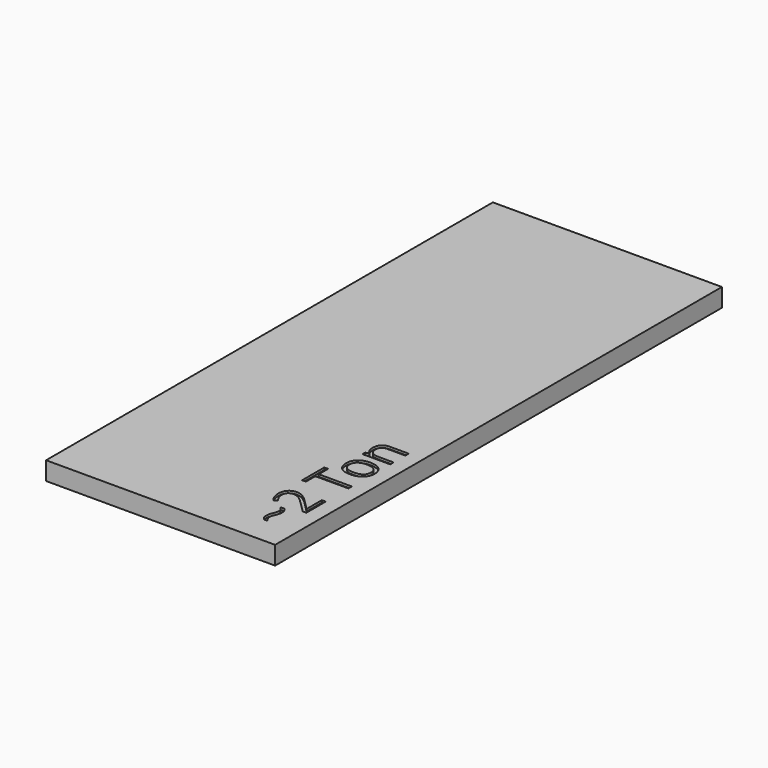
from build123d import *

# Parameters (mm, degrees)
F0_W         = 2500
F0_H         = 6096
F0_TEXT_SIZE = 565.0795168347
F1_DEPTH     = 200
F2_DEPTH     = 25


# Not quite as in the source:
# - Text() gives the source's letters only with a copy of the font that has no kerning and outlines rounded to 1/6400 em; it was checked with that copy


with BuildPart() as f1:
    # F0 (on Top) → F1 (new body)
    with BuildSketch(Plane.XY):
        Rectangle(F0_W, F0_H)
        with BuildLine():
            add(Edge.make_bspline(
                [(894.5491941284, -2651.680302651), (891.2381813344, -2664.1297107562), (891.2381813344, -2677.3737619321)],
                knots=[0, 0, 0, 1, 1, 1], degree=2))
            add(Edge.make_bspline(
                [(891.2381813344, -2677.3737619321), (891.2381813344, -2691.9422182254), (900.4648703202, -2709.4685126148)],
                knots=[0, 0, 0, 1, 1, 1], degree=2))
            add(Edge.make_bspline(
                [(900.4648703202, -2709.4685126148), (909.691559306, -2726.9948070041), (924.6131902975, -2741.9164379955)],
                knots=[0, 0, 0, 1, 1, 1], degree=2))
            Line((924.6131902975, -2741.9164379955), (882.9385759309, -2741.9164379955))
            add(Edge.make_bspline(
                [(882.9385759309, -2741.9164379955), (852.8304329245, -2714.2805178753), (852.8304329245, -2674.5483643479)],
                knots=[0, 0, 0, 1, 1, 1], degree=2))
            add(Edge.make_bspline(
                [(852.8304329245, -2674.5483643479), (852.8304329245, -2655.8301053527), (856.7153546028, -2640.2462718025)],
                knots=[0, 0, 0, 1, 1, 1], degree=2))
            add(Edge.make_bspline(
                [(856.7153546028, -2640.2462718025), (860.600276281, -2624.6624382523), (871.1072235472, -2600.1167967398)],
                knots=[0, 0, 0, 1, 1, 1], degree=2))
            add(Edge.make_bspline(
                [(871.1072235472, -2600.1167967398), (878.7887732291, -2581.8400061172), (882.5412543956, -2568.3310739179)],
                knots=[0, 0, 0, 1, 1, 1], degree=2))
            add(Edge.make_bspline(
                [(882.5412543956, -2568.3310739179), (886.2937355621, -2554.8221417185), (886.2937355621, -2541.8429715662)],
                knots=[0, 0, 0, 1, 1, 1], degree=2))
            add(Edge.make_bspline(
                [(886.2937355621, -2541.8429715662), (886.2937355621, -2527.0096342493), (877.4643681116, -2509.3508993482)],
                knots=[0, 0, 0, 1, 1, 1], degree=2))
            add(Edge.make_bspline(
                [(877.4643681116, -2509.3508993482), (868.635000661, -2491.6921644472), (852.8304329245, -2476.7705334557)],
                knots=[0, 0, 0, 1, 1, 1], degree=2))
            Line((852.8304329245, -2476.7705334557), (894.2401662676, -2476.7705334557))
            add(Edge.make_bspline(
                [(894.2401662676, -2476.7705334557), (924.6131902975, -2504.936215623), (924.6131902975, -2544.0503134289)],
                knots=[0, 0, 0, 1, 1, 1], degree=2))
            add(Edge.make_bspline(
                [(924.6131902975, -2544.0503134289), (924.6131902975, -2563.9163901926), (920.0660660604, -2581.3102440702)],
                knots=[0, 0, 0, 1, 1, 1], degree=2))
            add(Edge.make_bspline(
                [(920.0660660604, -2581.3102440702), (915.5189418234, -2598.7040979477), (906.6895743729, -2618.5701747114)],
                knots=[0, 0, 0, 1, 1, 1], degree=2))
            add(Edge.make_bspline(
                [(906.6895743729, -2618.5701747114), (897.8602069223, -2639.2308945457), (894.5491941284, -2651.680302651)],
                knots=[0, 0, 0, 1, 1, 1], degree=2))
        make_face(mode=Mode.SUBTRACT)
        with BuildLine():
            Line((1045.4872306954, -2154.7635025345), (1087.9564881325, -2154.7635025345))
            Line((1087.9564881325, -2154.7635025345), (1087.9564881325, -2419.9094070743))
            Line((1087.9564881325, -2419.9094070743), (1048.4892156286, -2419.9094070743))
            Line((1048.4892156286, -2419.9094070743), (941.7421631515, -2313.6921166442))
            add(Edge.make_bspline(
                [(941.7421631515, -2313.6921166442), (892.562586452, -2265.1305956663), (871.5928387569, -2249.6792026278)],
                knots=[0, 0, 0, 1, 1, 1], degree=2))
            add(Edge.make_bspline(
                [(871.5928387569, -2249.6792026278), (850.6230910619, -2234.2278095894), (830.7570142982, -2226.5021130701)],
                knots=[0, 0, 0, 1, 1, 1], degree=2))
            add(Edge.make_bspline(
                [(830.7570142982, -2226.5021130701), (810.8909375345, -2218.7764165509), (788.0228758376, -2218.7764165509)],
                knots=[0, 0, 0, 1, 1, 1], degree=2))
            add(Edge.make_bspline(
                [(788.0228758376, -2218.7764165509), (755.7073909686, -2218.7764165509), (736.8125446244, -2238.3776122911)],
                knots=[0, 0, 0, 1, 1, 1], degree=2))
            add(Edge.make_bspline(
                [(736.8125446244, -2238.3776122911), (717.9176982803, -2257.9788080313), (717.9176982803, -2292.7665157864)],
                knots=[0, 0, 0, 1, 1, 1], degree=2))
            add(Edge.make_bspline(
                [(717.9176982803, -2292.7665157864), (717.9176982803, -2317.841919346), (726.2173036838, -2340.3568063449)],
                knots=[0, 0, 0, 1, 1, 1], degree=2))
            add(Edge.make_bspline(
                [(726.2173036838, -2340.3568063449), (734.5169090873, -2362.8716933438), (756.3254466901, -2390.4193197894)],
                knots=[0, 0, 0, 1, 1, 1], degree=2))
            Line((756.3254466901, -2390.4193197894), (725.1577795897, -2414.7000802784))
            add(Edge.make_bspline(
                [(725.1577795897, -2414.7000802784), (678.8036004744, -2358.9867716655), (678.8036004744, -2293.2962778335)],
                knots=[0, 0, 0, 1, 1, 1], degree=2))
            add(Edge.make_bspline(
                [(678.8036004744, -2293.2962778335), (678.8036004744, -2236.435151452), (707.8963662239, -2204.1638134203)],
                knots=[0, 0, 0, 1, 1, 1], degree=2))
            add(Edge.make_bspline(
                [(707.8963662239, -2204.1638134203), (736.9891319734, -2171.8924753885), (786.0804149984, -2171.8924753885)],
                knots=[0, 0, 0, 1, 1, 1], degree=2))
            add(Edge.make_bspline(
                [(786.0804149984, -2171.8924753885), (824.4881634083, -2171.8924753885), (862.0129750731, -2193.4361319679)],
                knots=[0, 0, 0, 1, 1, 1], degree=2))
            add(Edge.make_bspline(
                [(862.0129750731, -2193.4361319679), (899.5377867379, -2214.9797885472), (956.9286751664, -2273.9599631168)],
                knots=[0, 0, 0, 1, 1, 1], degree=2))
            Line((956.9286751664, -2273.9599631168), (1043.2798888327, -2362.2536376222))
            Line((1043.2798888327, -2362.2536376222), (1045.4872306954, -2362.2536376222))
            Line((1045.4872306954, -2362.2536376222), (1045.4872306954, -2154.7635025345))
        make_face(mode=Mode.SUBTRACT)
        Polygon((726.2173036838, -1798.0570575326), (1087.9564881325, -1798.0570575326), (1087.9564881325, -1844.940998695), (726.2173036838, -1844.940998695), (726.2173036838, -1972.7019457043), (684.5426893172, -1972.7019457043), (684.5426893172, -1670.2961105232), (726.2173036838, -1670.2961105232), align=None, mode=Mode.SUBTRACT)
        with BuildLine():
            add(Edge.make_bspline(
                [(822.2366747084, -1392.83323839), (864.4851979593, -1355.4408672369), (936.4445426812, -1355.4408672369)],
                knots=[0, 0, 0, 1, 1, 1], degree=2))
            add(Edge.make_bspline(
                [(936.4445426812, -1355.4408672369), (1010.4346419167, -1355.4408672369), (1051.9768157715, -1392.656651041)],
                knots=[0, 0, 0, 1, 1, 1], degree=2))
            add(Edge.make_bspline(
                [(1051.9768157715, -1392.656651041), (1093.5189896263, -1429.872434845), (1093.5189896263, -1495.562928677)],
                knots=[0, 0, 0, 1, 1, 1], degree=2))
            add(Edge.make_bspline(
                [(1093.5189896263, -1495.562928677), (1093.5189896263, -1536.1780189495), (1074.4475559331, -1567.6105670734)],
                knots=[0, 0, 0, 1, 1, 1], degree=2))
            add(Edge.make_bspline(
                [(1074.4475559331, -1567.6105670734), (1055.37612224, -1599.0431151974), (1019.7937714143, -1616.1720880514)],
                knots=[0, 0, 0, 1, 1, 1], degree=2))
            add(Edge.make_bspline(
                [(1019.7937714143, -1616.1720880514), (984.2114205886, -1633.3010609055), (936.4445426812, -1633.3010609055)],
                knots=[0, 0, 0, 1, 1, 1], degree=2))
            add(Edge.make_bspline(
                [(936.4445426812, -1633.3010609055), (862.5427371201, -1633.3010609055), (821.2654442889, -1596.3060112877)],
                knots=[0, 0, 0, 1, 1, 1], degree=2))
            add(Edge.make_bspline(
                [(821.2654442889, -1596.3060112877), (779.9881514576, -1559.3109616699), (779.9881514576, -1493.6204678379)],
                knots=[0, 0, 0, 1, 1, 1], degree=2))
            add(Edge.make_bspline(
                [(779.9881514576, -1493.6204678379), (779.9881514576, -1430.225609543), (822.2366747084, -1392.83323839)],
                knots=[0, 0, 0, 1, 1, 1], degree=2))
        make_face(mode=Mode.SUBTRACT)
        with BuildLine():
            Line((1087.9564881325, -1022.308833328), (1087.9564881325, -1068.1332503963))
            Line((1087.9564881325, -1068.1332503963), (892.2977054285, -1068.1332503963))
            add(Edge.make_bspline(
                [(892.2977054285, -1068.1332503963), (855.3909494852, -1068.1332503963), (837.1583056998, -1084.9531953896)],
                knots=[0, 0, 0, 1, 1, 1], degree=2))
            add(Edge.make_bspline(
                [(837.1583056998, -1084.9531953896), (818.9256619145, -1101.7731403828), (818.9256619145, -1137.7086659066)],
                knots=[0, 0, 0, 1, 1, 1], degree=2))
            add(Edge.make_bspline(
                [(818.9256619145, -1137.7086659066), (818.9256619145, -1185.122369116), (844.5749743583, -1207.1957877423)],
                knots=[0, 0, 0, 1, 1, 1], degree=2))
            add(Edge.make_bspline(
                [(844.5749743583, -1207.1957877423), (870.2242868021, -1229.2692063687), (929.2927550462, -1229.2692063687)],
                knots=[0, 0, 0, 1, 1, 1], degree=2))
            Line((929.2927550462, -1229.2692063687), (1087.9564881325, -1229.2692063687))
            Line((1087.9564881325, -1229.2692063687), (1087.9564881325, -1275.093623437))
            Line((1087.9564881325, -1275.093623437), (785.5506529514, -1275.093623437))
            Line((785.5506529514, -1275.093623437), (785.5506529514, -1237.8336927957))
            Line((785.5506529514, -1237.8336927957), (826.9603862945, -1230.4170241372))
            Line((826.9603862945, -1230.4170241372), (826.9603862945, -1228.2096822746))
            add(Edge.make_bspline(
                [(826.9603862945, -1228.2096822746), (804.6220866446, -1214.0826943537), (792.3051190511, -1188.6982629334)],
                knots=[0, 0, 0, 1, 1, 1], degree=2))
            add(Edge.make_bspline(
                [(792.3051190511, -1188.6982629334), (779.9881514576, -1163.3138315131), (779.9881514576, -1132.1461644127)],
                knots=[0, 0, 0, 1, 1, 1], degree=2))
            add(Edge.make_bspline(
                [(779.9881514576, -1132.1461644127), (779.9881514576, -1077.4923798939), (806.3438132974, -1049.9006066109)],
                knots=[0, 0, 0, 1, 1, 1], degree=2))
            add(Edge.make_bspline(
                [(806.3438132974, -1049.9006066109), (832.6994751373, -1022.308833328), (890.7084192874, -1022.308833328)],
                knots=[0, 0, 0, 1, 1, 1], degree=2))
            Line((890.7084192874, -1022.308833328), (1087.9564881325, -1022.308833328))
        make_face(mode=Mode.SUBTRACT)
        with BuildLine():
            add(Edge.make_bspline(
                [(848.4598960365, -1562.8868554874), (877.9941301586, -1585.7990640216), (936.4445426812, -1585.7990640216)],
                knots=[0, 0, 0, 1, 1, 1], degree=2))
            add(Edge.make_bspline(
                [(936.4445426812, -1585.7990640216), (994.4534868312, -1585.7990640216), (1024.7823640238, -1562.6219744639)],
                knots=[0, 0, 0, 1, 1, 1], degree=2))
            add(Edge.make_bspline(
                [(1024.7823640238, -1562.6219744639), (1055.1112412165, -1539.4448849062), (1055.1112412165, -1494.503404583)],
                knots=[0, 0, 0, 1, 1, 1], degree=2))
            add(Edge.make_bspline(
                [(1055.1112412165, -1494.503404583), (1055.1112412165, -1449.4736305852), (1024.9148045356, -1426.1641005158)],
                knots=[0, 0, 0, 1, 1, 1], degree=2))
            add(Edge.make_bspline(
                [(1024.9148045356, -1426.1641005158), (994.7183678548, -1402.8545704463), (936.4445426812, -1402.8545704463)],
                knots=[0, 0, 0, 1, 1, 1], degree=2))
            add(Edge.make_bspline(
                [(936.4445426812, -1402.8545704463), (878.7887732291, -1402.8545704463), (848.8572175718, -1426.1641005158)],
                knots=[0, 0, 0, 1, 1, 1], degree=2))
            add(Edge.make_bspline(
                [(848.8572175718, -1426.1641005158), (818.9256619145, -1449.4736305852), (818.9256619145, -1495.03316663)],
                knots=[0, 0, 0, 1, 1, 1], degree=2))
            add(Edge.make_bspline(
                [(818.9256619145, -1495.03316663), (818.9256619145, -1539.9746469532), (848.4598960365, -1562.8868554874)],
                knots=[0, 0, 0, 1, 1, 1], degree=2))
        make_face()
        with Locations(Location((1087.9564881325, -2770.6118822098), (0, 0, 90))):
            Text('~2 Ton', F0_TEXT_SIZE, font='Open Sans', text_align=(TextAlign.LEFT, TextAlign.BOTTOM))
    extrude(amount=-F1_DEPTH)

    # F0 (on Top) → F2 (cut)
    with BuildSketch(Plane.XY):
        with Locations(Location((1087.9564881325, -2770.6118822098), (0, 0, 90))):
            Text('~2 Ton', F0_TEXT_SIZE, font='Open Sans', text_align=(TextAlign.LEFT, TextAlign.BOTTOM))
    extrude(amount=-F2_DEPTH, mode=Mode.SUBTRACT)


solid = f1.part
